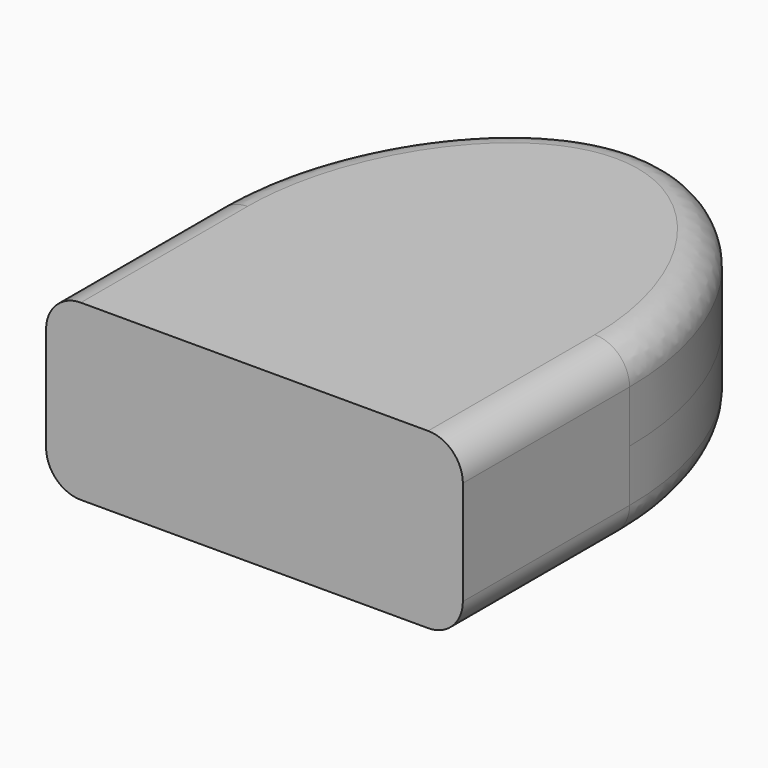
from build123d import *

# Parameters (mm, degrees)
F1_DEPTH = 12.5
F2_R     = 5
F3_W     = 43
F3_H     = 32
F4_DEPTH = 1


# Not quite as in the source:
# - ends of sketch curves that miss each other by under 0.0002 mm in the source are joined


with BuildPart() as f1:
    # F0 (on Top) → F1 (new body, symmetric)
    with BuildSketch(Plane.XY):
        with BuildLine():
            Line((-30, -8.0950134536), (-30, -38.0950163982))
            Line((-30, -38.0950163982), (0, -38.0950163982))
            ThreePointArc((0, -38.0950163982), (-21.2132044767, -29.3082187928), (-30, -8.0950134536))
        make_face()
        with BuildLine():
            ThreePointArc((30, -8.0950163982), (21.2132034356, -29.3082198338), (0, -38.0950163982))
            Line((0, -38.0950163982), (30, -38.0950163982))
            Line((30, -38.0950163982), (30, -8.0950163982))
        make_face()
        with BuildLine():
            ThreePointArc((-30, -8.0950134536), (-21.2132044767, -29.3082187928), (0, -38.0950163982))
            ThreePointArc((0, -38.0950163982), (21.2132034356, -29.3082198338), (30, -8.0950163982))
            ThreePointArc((30, -8.0950163982), (1.4723e-06, 21.9049836018), (-30, -8.0950134536))
        make_face()
        with BuildLine():
            add(Edge.make_bspline(
                [(0, 31.9049836018), (-16.629870981, 31.9049836018), (-30, 11.955471457), (-30, -8.0950134536)],
                knots=[0, 0, 0, 0, 49.9999976443, 49.9999976443, 49.9999976443, 49.9999976443], degree=3))
            ThreePointArc((-30, -8.0950134536), (1.4723e-06, 21.9049836018), (30, -8.0950163982))
            add(Edge.make_bspline(
                [(0, 31.9049836018), (16.629870981, 31.9049836018), (30, 11.955471457), (30, -8.0950163982)],
                knots=[0, 0, 0, 0, 49.9999976443, 49.9999976443, 49.9999976443, 49.9999976443], degree=3))
        make_face()
    extrude(amount=F1_DEPTH, both=True)

    # F2
    f2_edges = [f1.edges().sort_by_distance(p)[0] for p in [
        (30, -23.095016, -12.5),
        (30, -23.095016, 12.5),
        (-30, -23.095015, 12.5),
        (-30, -23.095015, -12.5),
    ]]
    fillet(f2_edges, radius=F2_R)

    # F3 (on face) → F4 (cut)
    with BuildSketch(Plane(origin=(0, 0, -12.5), x_dir=(1, 0, 0), z_dir=(0, 0, -1))):
        with Locations((0, 20)):
            Rectangle(F3_W, F3_H)
    extrude(amount=-F4_DEPTH, mode=Mode.SUBTRACT)


solid = f1.part
